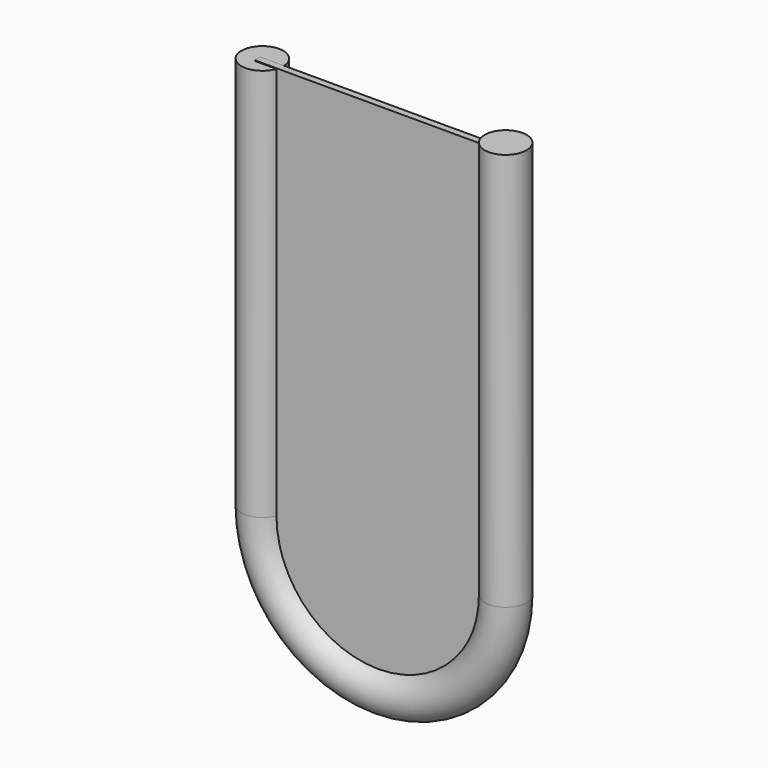
from build123d import *

# Parameters (mm, degrees)
F2_R     = 3.7933293271
F4_W     = 44.7215028107
F4_H     = 71.540701203
F5_DEPTH = 1.27


# Not quite as in the source:
# - a feature of the source that left no trace in its solid (it failed there, or was rolled back) is left out


with BuildPart() as f3:
    # F3: sweep along a path in F0
    with BuildLine(Plane.XZ) as f3_path:
        Line((-44.6055270731, 57.5704574585), (-44.6055270731, -13.7366456911))
        ThreePointArc((-44.6055270731, -13.7366456911), (-22.3027635366, -36.0394092277), (0, -13.7366456911))
        Line((0, -13.7366456911), (0, 58.4965236485))
    # F2 (on line) → F3 (sweep)
    with BuildSketch(Plane(origin=(0, 0, 57.5704574585), x_dir=(1, 0, 0), z_dir=(0, 0, -1))):
        with Locations((-44.3615987897, 0)):
            Circle(F2_R)
    sweep(path=f3_path.line)

    # F4 (on Front) → F5 (join)
    with BuildSketch(Plane.XZ):
        with Locations((-22.3607514054, 21.9205492176)):
            Rectangle(F4_W, F4_H)
        with BuildLine():
            Line((0, -13.8498013839), (-44.7215028107, -13.8498013839))
            ThreePointArc((-44.7215028107, -13.8498013839), (-22.3607514054, -36.2105527893), (0, -13.8498013839))
        make_face()
    extrude(amount=F5_DEPTH)


solid = f3.part
